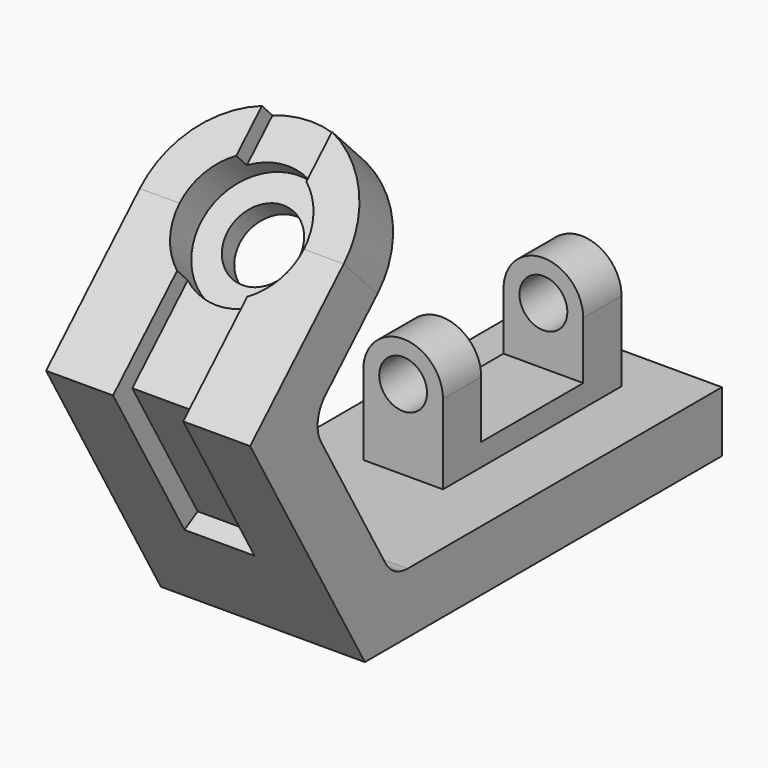
from build123d import *

# Parameters (mm, degrees)
F1_DEPTH  = 64
F4_DEPTH  = 19
F6_DEPTH  = 6
F8_DEPTH  = 6
F9_R      = 19.5
F10_DEPTH = 12
F11_R     = 11.1871907606
F12_DEPTH = 25
F13_W     = 12.5
F13_H     = 70
F14_DEPTH = 25
F16_DEPTH = 70
F17_R     = 7.5
F18_DEPTH = 70
F19_W     = 40
F19_H     = 38.5815599019
F20_DEPTH = 44.501


with BuildPart() as f1:
    # F0 (on Right) → F1 (new body)
    with BuildSketch(Plane.YZ):
        with BuildLine():
            Line((-54.1868201462, -31.8179203436), (85.8131798538, -31.8179203436))
            Line((85.8131798538, -31.8179203436), (85.8131798538, -12.8179203436))
            Line((85.8131798538, -12.8179203436), (-37.4436623397, -12.8179203436))
            ThreePointArc((-37.4436623397, -12.8179203436), (-42.4436623397, -11.4781743814), (-46.1039163775, -7.8179203436))
            Line((-46.1039163775, -7.8179203436), (-71.3920766998, 35.9824581646))
            ThreePointArc((-71.3920766998, 35.9824581646), (-72.6338098814, 42.3791145671), (-69.671246979, 48.1827630296))
            Line((-69.671246979, 48.1827630296), (-49.2803591326, 67.8348507705))
            Line((-49.2803591326, 67.8348507705), (-62.4652653349, 81.5154300139))
            Line((-62.4652653349, 81.5154300139), (-99.1868201462, 46.124365997))
            Line((-99.1868201462, 46.124365997), (-54.1868201462, -31.8179203436))
        make_face()
    extrude(amount=F1_DEPTH)

    # F3 (on face) → F4 (join)
    with BuildSketch(Plane(origin=(0, -70.8105053198, 73.4725537235), x_dir=(1, 0, 0), z_dir=(0, -0.6939424317, 0.7200304865))):
        with BuildLine():
            Line((0, 11.5901203371), (64, 11.5901203371))
            ThreePointArc((64, 11.5901203371), (32, 43.5901203371), (0, 11.5901203371))
        make_face()
    extrude(amount=-F4_DEPTH)

    # F2 (on face) → F6 (cut)
    with BuildSketch(Plane(origin=(0, -54.4176787662, -31.4180614843), x_dir=(1, 0, 0), z_dir=(0, -0.8660254038, -0.5))):
        Polygon((21, 113.3266016841), (21, 89.53828276), (21, 33.53828276), (43, 33.53828276), (43, 89.53828276), (43, 113.3266016841), align=None)
    extrude(amount=-F6_DEPTH, mode=Mode.SUBTRACT)

    # F7 (on face) → F8 (cut)
    with BuildSketch(Plane(origin=(0, -70.8105053198, 73.4725537235), x_dir=(1, 0, 0), z_dir=(0, -0.6939424317, 0.7200304865))):
        with BuildLine():
            Line((21, 41.6400787397), (21, -39.4098796629))
            Line((21, -39.4098796629), (43, -39.4098796629))
            Line((43, -39.4098796629), (43, 41.6400787397))
            ThreePointArc((43, 41.6400787397), (32, 43.5901203371), (21, 41.6400787397))
        make_face()
    extrude(amount=-F8_DEPTH, mode=Mode.SUBTRACT)

    # F9 (on face) → F10 (cut)
    with BuildSketch(Plane(origin=(0, -70.8105053198, 73.4725537235), x_dir=(1, 0, 0), z_dir=(0, -0.6939424317, 0.7200304865))):
        with Locations((32, 11.5901203371)):
            Circle(F9_R)
    extrude(amount=-F10_DEPTH, mode=Mode.SUBTRACT)

    # F11 (on face) → F12 (cut)
    with BuildSketch(Plane(origin=(0, -70.8105053198, 73.4725537235), x_dir=(1, 0, 0), z_dir=(0, -0.6939424317, 0.7200304865))):
        with Locations((32, 11.5901203371)):
            Circle(F11_R)
    extrude(amount=-F12_DEPTH, mode=Mode.SUBTRACT)

    # F13 (on face) → F14 (join)
    with BuildSketch(Plane.XY.offset(-12.8179203436)):
        with Locations((25.75, 35.8131798538)):
            Rectangle(F13_W, F13_H)
        with Locations((38.25, 35.8131798538)):
            Rectangle(F13_W, F13_H)
    extrude(amount=F14_DEPTH)

    # F15 (on face) → F16 (join, through all)
    with BuildSketch(Plane(origin=(0, 70.8131798538, 0), x_dir=(-1, 0, 0), z_dir=(0, 1, 0))):
        with BuildLine():
            Line((-44.5, 12.1820796564), (-19.5, 12.1820796564))
            ThreePointArc((-19.5, 12.1820796564), (-32, 24.6820796564), (-44.5, 12.1820796564))
        make_face()
    extrude(amount=-F16_DEPTH)

    # F17 (on face) → F18 (cut, through all)
    with BuildSketch(Plane(origin=(0, 70.8131798538, 0), x_dir=(-1, 0, 0), z_dir=(0, 1, 0))):
        with Locations((-32, 12.1820796564)):
            Circle(F17_R)
    extrude(amount=-F18_DEPTH, mode=Mode.SUBTRACT)

    # F19 (on face) → F20 (cut, through all)
    with BuildSketch(Plane.YZ.offset(44.5)):
        with Locations((35.8131798538, 13.4728596074)):
            Rectangle(F19_W, F19_H)
    extrude(amount=-F20_DEPTH, mode=Mode.SUBTRACT)


solid = f1.part
